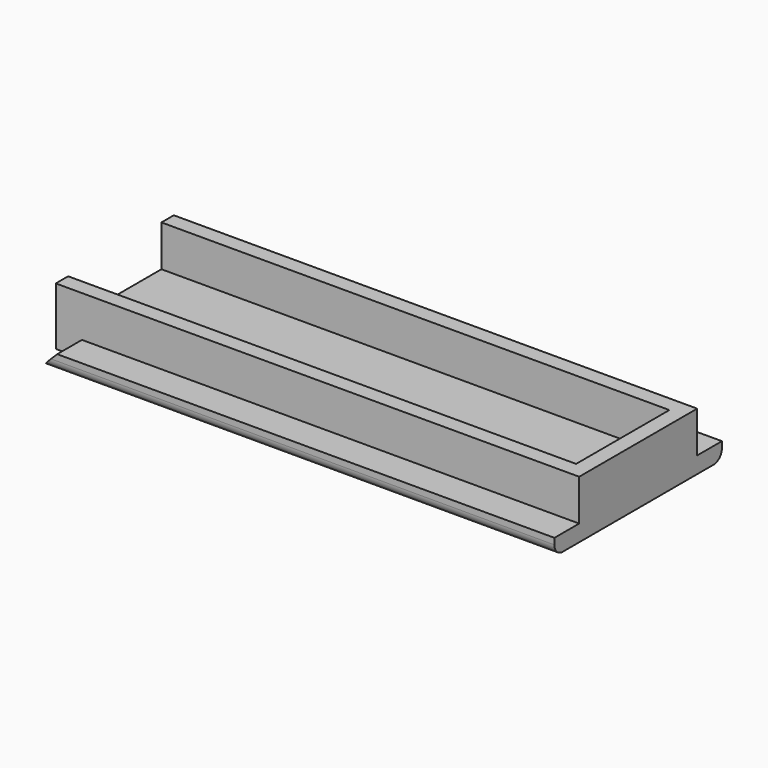
from build123d import *

# Parameters (mm, degrees)
F0_W        = 50.8
F0_H        = 20.32
F1_DEPTH    = 1.6
F2_W        = 1.5
F2_H        = 11.32
F3_DEPTH    = 4
F4_R        = 1
F5_T1_DEPTH = 9.5320747894
F5_T3_DEPTH = 9.5320747894


# Not quite as in the source:
# - a fillet or chamfer that OpenCascade refuses, or shapes differently, is made with other operations: its cross-section is extruded or revolved along the edge and cut away or added


with BuildPart() as f1:
    # F0 (on Top) → F1 (new body)
    with BuildSketch(Plane.XY):
        Rectangle(F0_W, F0_H)
    extrude(amount=F1_DEPTH)

    # F2 (on face) → F3 (join)
    with BuildSketch(Plane.XY.offset(1.6)):
        Polygon((25.4, 7.16), (-25.4, 7.16), (-25.4, 5.66), (23.9, 5.66), (25.4, 5.66), align=None)
        with Locations((24.65, 0)):
            Rectangle(F2_W, F2_H)
        Polygon((25.4, -7.16), (25.4, -5.66), (23.9, -5.66), (-25.4, -5.66), (-25.4, -7.16), align=None)
    extrude(amount=F3_DEPTH)

    # F4
    f4_edges = [f1.edges().sort_by_distance(p)[0] for p in [
        (0, -10.16, 0),
        (0, 10.16, 0),
    ]]
    fillet(f4_edges, radius=F4_R)

    # F5: chamfer of 2.54 on 2 edges, made by hand

    # F5_s2 → F5_t1 (cut)
    with BuildSketch(Plane.XZ.offset(-16.6920747894)):
        Polygon((-22.86, 1.6), (-25.4, -0.94), (-25.4, 1.6), align=None)
    extrude(amount=F5_T1_DEPTH, mode=Mode.SUBTRACT)

    # F5_s4 → F5_t3 (cut)
    with BuildSketch(Plane.XZ.offset(7.16)):
        Polygon((-25.4, -0.94), (-22.86, 1.6), (-25.4, 1.6), align=None)
    extrude(amount=F5_T3_DEPTH, mode=Mode.SUBTRACT)


solid = f1.part
